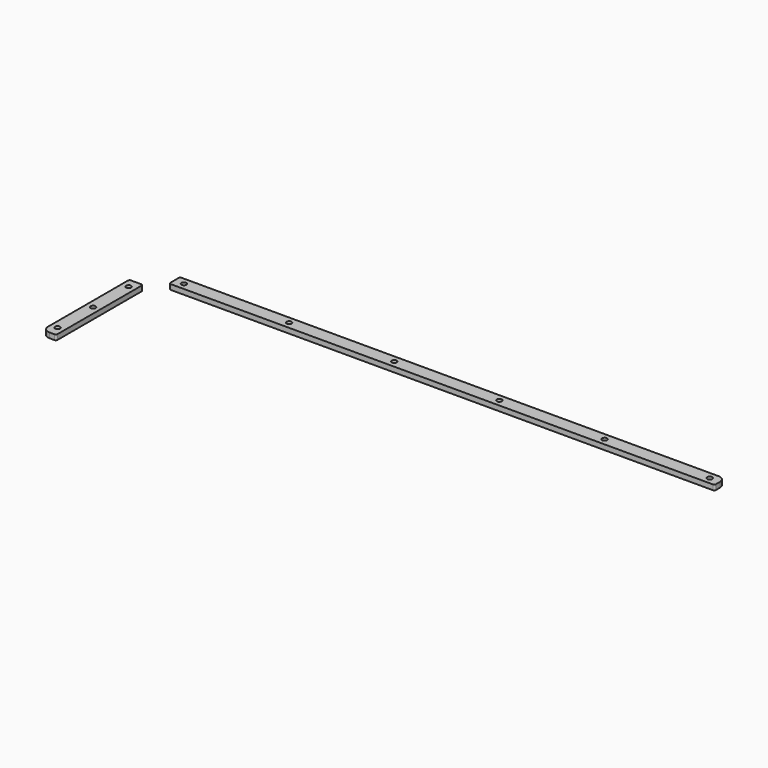
from build123d import *

# Parameters (mm, degrees)
F0_R     = 2.38125
F1_DEPTH = 4.7625
F4_W     = 13.49375
F4_H     = 13.49375
F4_W_2   = 139.7
F4_H_2   = 38.1
F5_DEPTH = 4.7635
F7_DEPTH = 4.7625


# Not quite as in the source:
# - a feature of the source that left no trace in its solid (it failed there, or was rolled back) is left out


with BuildPart() as f1:
    # F0 (on Top) → F1 (new body)
    with BuildSketch(Plane.XY):
        with BuildLine():
            ThreePointArc((0, 6.35), (1.8598719395, 1.8598719395), (6.35, 0))
            Line((6.35, 0), (527.05, 0))
            ThreePointArc((527.05, 0), (531.5401280605, 1.8598719395), (533.4, 6.35))
            Line((533.4, 6.35), (533.4, 120.65))
            ThreePointArc((533.4, 120.65), (531.5401280605, 125.1401280605), (527.05, 127))
            Line((527.05, 127), (400.05, 127))
            ThreePointArc((400.05, 127), (395.5598719395, 128.8598719395), (393.7, 133.35))
            Line((393.7, 133.35), (393.7, 152.4))
            ThreePointArc((393.7, 152.4), (391.8401280605, 156.8901280605), (387.35, 158.75))
            Line((387.35, 158.75), (273.05, 158.75))
            ThreePointArc((273.05, 158.75), (268.5598719395, 156.8901280605), (266.7, 152.4))
            Line((266.7, 152.4), (266.7, 133.35))
            ThreePointArc((266.7, 133.35), (264.8401280605, 128.8598719395), (260.35, 127))
            Line((260.35, 127), (6.35, 127))
            ThreePointArc((6.35, 127), (1.8598719395, 125.1401280605), (0, 120.65))
            Line((0, 120.65), (0, 6.35))
        make_face()
        with Locations((6.35, 9.525)):
            Circle(F0_R, mode=Mode.SUBTRACT)
        with Locations((228.6, 31.75)):
            Circle(F0_R, mode=Mode.SUBTRACT)
        with Locations((6.35, 50.8)):
            Circle(F0_R, mode=Mode.SUBTRACT)
        with Locations((457.2, 31.75)):
            Circle(F0_R, mode=Mode.SUBTRACT)
        with Locations((6.35, 92.075)):
            Circle(F0_R, mode=Mode.SUBTRACT)
        with Locations((228.6, 95.25)):
            Circle(F0_R, mode=Mode.SUBTRACT)
        with Locations((34.925, 120.65)):
            Circle(F0_R, mode=Mode.SUBTRACT)
        with Locations((132.715, 120.65)):
            Circle(F0_R, mode=Mode.SUBTRACT)
        with Locations((230.505, 120.65)):
            Circle(F0_R, mode=Mode.SUBTRACT)
        with BuildLine():
            ThreePointArc((254, 107.95), (255.8598719395, 112.4401280605), (260.35, 114.3))
            Line((260.35, 114.3), (400.05, 114.3))
            ThreePointArc((400.05, 114.3), (404.5401280605, 112.4401280605), (406.4, 107.95))
            Line((406.4, 107.95), (406.4, 69.85))
            ThreePointArc((406.4, 69.85), (404.5401280605, 65.3598719395), (400.05, 63.5))
            Line((400.05, 63.5), (260.35, 63.5))
            ThreePointArc((260.35, 63.5), (255.8598719395, 65.3598719395), (254, 69.85))
            Line((254, 69.85), (254, 107.95))
        make_face(mode=Mode.SUBTRACT)
        with Locations((457.2, 95.25)):
            Circle(F0_R, mode=Mode.SUBTRACT)
        with Locations((328.295, 120.65)):
            Circle(F0_R, mode=Mode.SUBTRACT)
        with Locations((307.975, 147.6375)):
            Circle(F0_R, mode=Mode.SUBTRACT)
        with Locations((352.425, 147.6375)):
            Circle(F0_R, mode=Mode.SUBTRACT)
        with Locations((426.085, 120.65)):
            Circle(F0_R, mode=Mode.SUBTRACT)
        with Locations((523.875, 120.65)):
            Circle(F0_R, mode=Mode.SUBTRACT)
    extrude(amount=F1_DEPTH)

    # F4 (on face) → F5 (cut, through all)
    with BuildSketch(Plane.XY.offset(4.7625)):
        Polygon((26.19375, 127), (0, 127), (0, 100.80625), (12.7, 100.80625), (12.7, 114.3), (26.19375, 114.3), align=None)
        Polygon((533.4, 114.3), (26.19375, 114.3), (26.19375, 100.80625), (12.7, 100.80625), (12.7, 0), (533.4, 0), align=None)
        with Locations((19.446875, 107.553125)):
            Rectangle(F4_W, F4_H)
        with Locations((330.2, 146.05)):
            Rectangle(F4_W_2, F4_H_2)
    extrude(amount=-F5_DEPTH, mode=Mode.SUBTRACT)

    # F6 (on face) → F7 (cut, through all)
    with BuildSketch(Plane.XY.offset(4.7625)):
        with BuildLine():
            Line((12.7, 99.21875), (12.7, 100.80625))
            Line((12.7, 100.80625), (11.1125, 100.80625))
            ThreePointArc((11.1125, 100.80625), (12.2350320151, 100.3412820151), (12.7, 99.21875))
        make_face()
        with BuildLine():
            Line((1.5875, 100.80625), (0, 100.80625))
            Line((0, 100.80625), (0, 99.21875))
            ThreePointArc((0, 99.21875), (0.4649679849, 100.3412820151), (1.5875, 100.80625))
        make_face()
        with BuildLine():
            ThreePointArc((12.7, 1.5875), (12.2350320151, 0.4649679849), (11.1125, 0))
            Line((11.1125, 0), (12.7, 0))
            Line((12.7, 0), (12.7, 1.5875))
        make_face()
        with BuildLine():
            ThreePointArc((26.19375, 125.4125), (26.6587179849, 126.5350320151), (27.78125, 127))
            Line((27.78125, 127), (26.19375, 127))
            Line((26.19375, 127), (26.19375, 125.4125))
        make_face()
        with BuildLine():
            Line((26.19375, 115.8875), (26.19375, 114.3))
            Line((26.19375, 114.3), (27.78125, 114.3))
            ThreePointArc((27.78125, 114.3), (26.6587179849, 114.7649679849), (26.19375, 115.8875))
        make_face()
        with BuildLine():
            Line((531.8125, 114.3), (533.4, 114.3))
            Line((533.4, 114.3), (533.4, 115.8875))
            ThreePointArc((533.4, 115.8875), (532.9350320151, 114.7649679849), (531.8125, 114.3))
        make_face()
    extrude(amount=-F7_DEPTH, mode=Mode.SUBTRACT)


solid = f1.part
